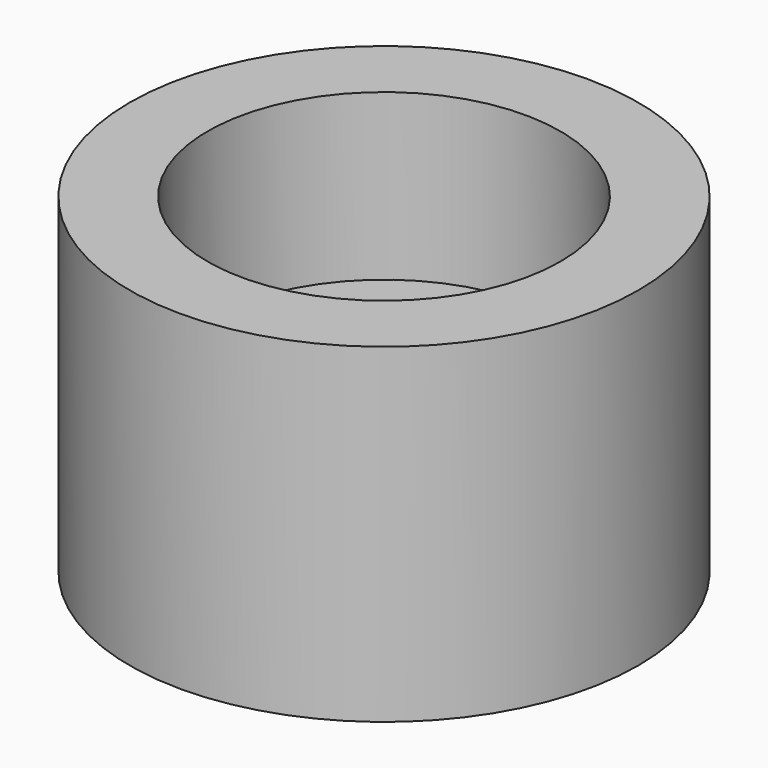
from build123d import *

# Parameters (mm, degrees)
F0_R     = 19.5560512616
F1_DEPTH = 25.4
F5_R     = 13.568481042
F6_DEPTH = 12.7


# Not quite as in the source:
# - the program builds the solid bodies; features that only make, move or delete a surface that nothing else refers to are left out


with BuildPart() as f1:
    # F0 (on Top) → F1 (new body)
    with BuildSketch(Plane.XY):
        Circle(F0_R)
    extrude(amount=F1_DEPTH)

    # F5 (on face) → F6 (cut)
    with BuildSketch(Plane.XY.offset(25.4)):
        Circle(F5_R)
    extrude(amount=-F6_DEPTH, mode=Mode.SUBTRACT)


solid = f1.part
